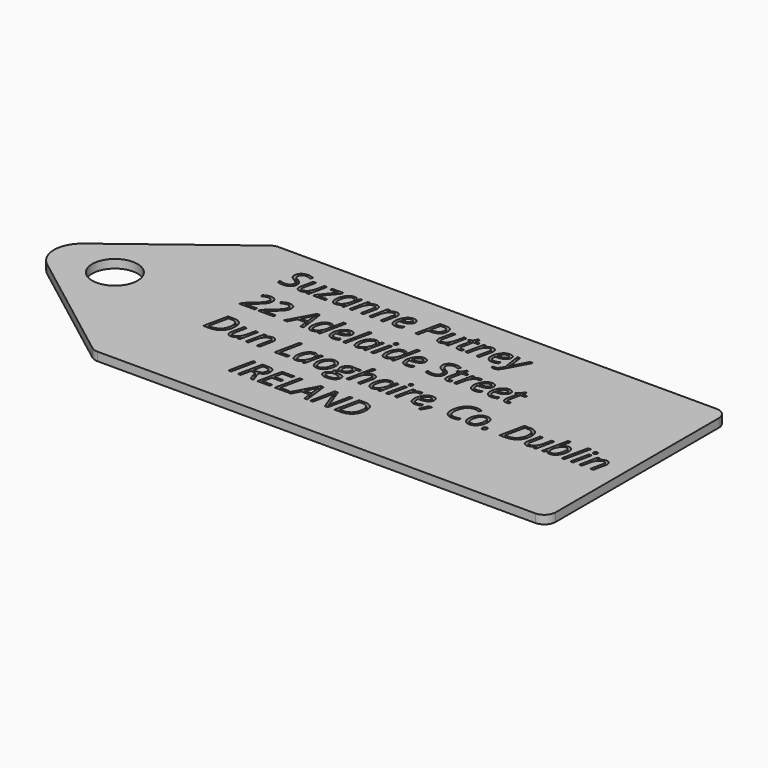
from build123d import *

# Parameters (mm, degrees)
F0_W         = 80
F0_H         = 40
F1_DEPTH     = 1.5
F2_TEXT_SIZE = 6.0665150038
F3_DEPTH     = 0.75
F5_DEPTH     = 1.5
F7_R         = 2
F8_R         = 4
F9_DEPTH     = 2


# Not quite as in the source:
# - Text() gives the source's letters only with a copy of the font that has no kerning and outlines rounded to 1/6400 em; it was checked with that copy


with BuildPart() as f1:
    # F0 (on Top) → F1 (new body)
    with BuildSketch(Plane.XY):
        with Locations((-9.0164969116, 7.607867457)):
            Rectangle(F0_W, F0_H)
    extrude(amount=F1_DEPTH)

    # F2 (on face) → F3 (cut)
    with BuildSketch(Plane.XY.offset(1.5)):
        with Locations((-42.0164969116, 19.2399766542)):
            Text('Suzanne Putney', F2_TEXT_SIZE, font='Open Sans', font_style=FontStyle.ITALIC, text_align=(TextAlign.LEFT, TextAlign.BOTTOM))
        with Locations((-42.0164969116, 10.9895162491)):
            Text('22 Adelaide Street', F2_TEXT_SIZE, font='Open Sans', font_style=FontStyle.ITALIC, text_align=(TextAlign.LEFT, TextAlign.BOTTOM))
        with Locations((-42.0164969116, 2.7390558439)):
            Text('Dun Laoghaire, Co. Dublin', F2_TEXT_SIZE, font='Open Sans', font_style=FontStyle.ITALIC, text_align=(TextAlign.LEFT, TextAlign.BOTTOM))
        with Locations((-30.9820748555, -5.5114045612)):
            Text('IRELAND', F2_TEXT_SIZE, font='Open Sans', font_style=FontStyle.ITALIC, text_align=(TextAlign.LEFT, TextAlign.BOTTOM))
    extrude(amount=-F3_DEPTH, mode=Mode.SUBTRACT)


with BuildPart() as f5:
    # F4 (on face) → F5 (new body)
    with BuildSketch(Plane.XY.offset(1.5)):
        with BuildLine():
            Line((-49.0164969116, -12.392132543), (-49.0164969116, 27.607867457))
            Line((-49.0164969116, 27.607867457), (-70.0456094388, 11.584959805))
            ThreePointArc((-70.0456094388, 11.584959805), (-72.0153064085, 7.607867457), (-70.0456094388, 3.630775109))
            Line((-70.0456094388, 3.630775109), (-49.0164969116, -12.392132543))
        make_face()
    extrude(amount=-F5_DEPTH)


with BuildPart() as f1_1:
    add(f1.part)

    # F6: union F5
    add(f5.part)

    # F7
    f7_edges = [f1_1.edges().sort_by_distance(p)[0] for p in [
        (-49.016497, 27.607867, 0.75),
        (30.983503, 27.607867, 0.75),
        (30.983503, -12.392133, 0.75),
        (-49.016497, -12.392133, 0.75),
    ]]
    fillet(f7_edges, radius=F7_R)

    # F8 (on face) → F9 (cut)
    with BuildSketch(Plane.XY.offset(1.5)):
        with Locations((-61.2635016441, 7.607867457)):
            Circle(F8_R)
    extrude(amount=-F9_DEPTH, mode=Mode.SUBTRACT)


solid = f1_1.part
